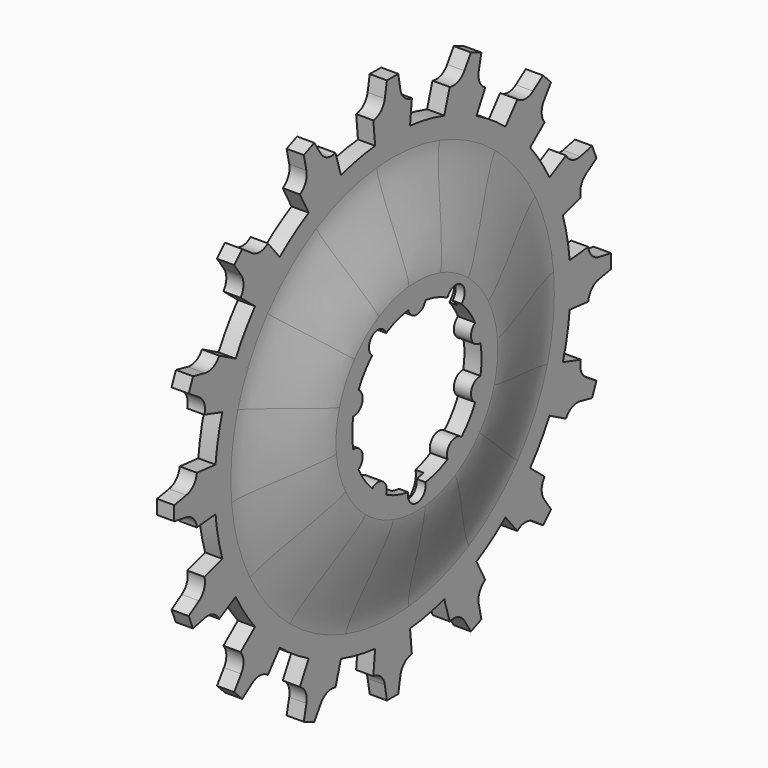
from build123d import *

# Parameters (mm, degrees)
F1_DEPTH       = 2.125
F4_DEPTH       = 4.251
F6_ANGLE_BACK  = 5.625
F6_ANGLE       = 22.5
F8_DEPTH       = 10.2510001
F9_COUNT       = 16
F10_R          = 2.75
F11_DEPTH      = 4.25
F12_COUNT      = 10
F13_R          = 2.75
F14_DEPTH      = 10.2510001
F15_R          = 5
F16_DEPTH      = 2
F16_DEPTH_BACK = 6.0010001


# Not quite as in the source:
# - the dataset's text gives a spline's control points without its knots; the knots are read off the source's solid


with BuildPart() as f1:
    # F0 (on Right) → F1 (new body, symmetric)
    with BuildSketch(Plane.YZ):
        with BuildLine():
            Line((-5.9579314387, 60.4918930546), (0, 0))
            Line((0, 0), (5.9579314387, 60.4918930546))
            ThreePointArc((5.9579314387, 60.4918930546), (3.6315945475, 61.5383054975), (2.410768988, 63.7780392506))
            Line((2.410768988, 63.7780392506), (1.7559163599, 67.4918930546))
            Line((1.7559163599, 67.4918930546), (-1.7559163599, 67.4918930546))
            Line((-1.7559163599, 67.4918930546), (-2.410768988, 63.7780392506))
            ThreePointArc((-2.410768988, 63.7780392506), (-3.6315945475, 61.5383054975), (-5.9579314387, 60.4918930546))
        make_face()
    extrude(amount=F1_DEPTH, both=True)

    # F3 (on face) → F4 (cut, through all)
    with BuildSketch(Plane.YZ.offset(2.125)):
        with BuildLine():
            Line((0, 0), (5.3909427181, 54.735159967))
            ThreePointArc((5.3909427181, 54.735159967), (0, 55), (-5.3909427181, 54.735159967))
            Line((-5.3909427181, 54.735159967), (0, 0))
        make_face()
        with BuildLine():
            ThreePointArc((-5.3909427181, 54.735159967), (-36.9357425166, -40.7523118945), (55, 0))
            ThreePointArc((55, 0), (40.7523118945, 36.9357425166), (5.3909427181, 54.735159967))
            Line((5.3909427181, 54.735159967), (0, 0))
            Line((0, 0), (-5.3909427181, 54.735159967))
        make_face()
    extrude(amount=-F4_DEPTH, mode=Mode.SUBTRACT)

    # F5 (on Front) → F6 (revolve)
    with BuildSketch(Plane.XZ, mode=Mode.PRIVATE) as f6_sk:
        with BuildLine():
            Line((2.125, 55), (-2.125, 55))
            Line((-2.125, 55), (-2.125, 50))
            add(Edge.make_bspline(
                [(-2.125, 50), (-2.125, 49.475), (-2.0513729162, 48.4735258484), (-1.8145131722, 46.9449385287), (-1.4788846464, 45.337822078), (-0.9257646602, 43.077276111), (-0.0776192793, 40.0515383237), (1.0576670714, 36.2673880676), (2.1723807207, 32.5515383237), (2.9648603398, 29.717901111), (3.4429903536, 27.759697078), (3.7050180778, 26.4957197787), (3.8548770838, 25.5047758484), (3.875, 25.1), (3.875, 25)],
                knots=[0, 0, 0, 0, 0.0625, 0.125, 0.1875, 0.25, 0.375, 0.5, 0.625, 0.75, 0.8125, 0.875, 0.9375, 1, 1, 1, 1], degree=3))
            Line((3.875, 25), (3.875, 0))
            Line((3.875, 0), (8.125, 0))
            Line((8.125, 0), (8.125, 25))
            add(Edge.make_bspline(
                [(2.125, 50), (2.125, 45), (8.125, 30), (8.125, 25)],
                knots=[0, 0, 0, 0, 25.7099202644, 25.7099202644, 25.7099202644, 25.7099202644], degree=3))
            Line((2.125, 50), (2.125, 55))
        make_face()
    revolve(f6_sk.sketch.rotate(Axis((21.9800565392, 0, 0), (-1, 0, 0)), -F6_ANGLE_BACK), axis=Axis((21.9800565392, 0, 0), (-1, 0, 0)), revolution_arc=F6_ANGLE)

    # F7 (on face) → F8 (cut, through all)
    with BuildSketch(Plane.YZ.offset(8.125)):
        with BuildLine():
            Line((0, 0), (5.8056935451, 19.1388067146))
            ThreePointArc((5.8056935451, 19.1388067146), (1.9603428066, 19.9036945334), (-1.9603428066, 19.9036945334))
            Line((-1.9603428066, 19.9036945334), (0, 0))
        make_face()
        with BuildLine():
            ThreePointArc((-1.9603428066, 19.9036945334), (-13.4311790969, -14.8190225071), (20, 0))
            ThreePointArc((20, 0), (16.0641506296, 11.9139860898), (5.8056935451, 19.1388067146))
            Line((5.8056935451, 19.1388067146), (0, 0))
            Line((0, 0), (-1.9603428066, 19.9036945334))
        make_face()
    extrude(amount=-F8_DEPTH, mode=Mode.SUBTRACT)

    # F9: F1 ×16 about axis
    f9_axis = Axis((21.9800565392, 0, 0), (1, 0, 0))


with BuildPart() as f1_1:
    add(f1.part)
    for i in range(1, F9_COUNT):
        add(f1.part.rotate(f9_axis, i * 360 / F9_COUNT))

    # F10 (on face) → F11 (join, through all)
    with BuildSketch(Plane.YZ.offset(8.125)):
        with Locations((0, -20.5)):
            Circle(F10_R)
    f11 = extrude(amount=-F11_DEPTH)

    # F12: F11 ×10 about axis
    f12_axis = Axis((21.9800565392, 0, 0), (1, 0, 0))
    for i in range(1, F12_COUNT):
        add(f11.rotate(f12_axis, i * 360 / F12_COUNT))

    # F13 (on face) → F14 (cut, through all)
    with BuildSketch(Plane.YZ.offset(8.125)):
        with Locations((0, -20.5)):
            Circle(F13_R)
        with Locations((-12.049597672, 16.5848483847)):
            Circle(F13_R)
        with Locations((12.049597672, 16.5848483847)):
            Circle(F13_R)
    extrude(amount=-F14_DEPTH, mode=Mode.SUBTRACT)

    # F15 (on face) → F16 (cut, two sides)
    with BuildSketch(Plane(origin=(3.875, 0, 0), x_dir=(0, -1, 0), z_dir=(-1, 0, 0))) as f16_sk:
        with Locations((-12.049597672, 16.5848483847)):
            Circle(F15_R)
        with Locations((12.049597672, 16.5848483847)):
            Circle(F15_R)
        with Locations((0, -20.5)):
            Circle(F15_R)
    extrude(amount=-F16_DEPTH, mode=Mode.SUBTRACT)
    extrude(f16_sk.sketch, amount=F16_DEPTH_BACK, mode=Mode.SUBTRACT)


solid = f1_1.part
